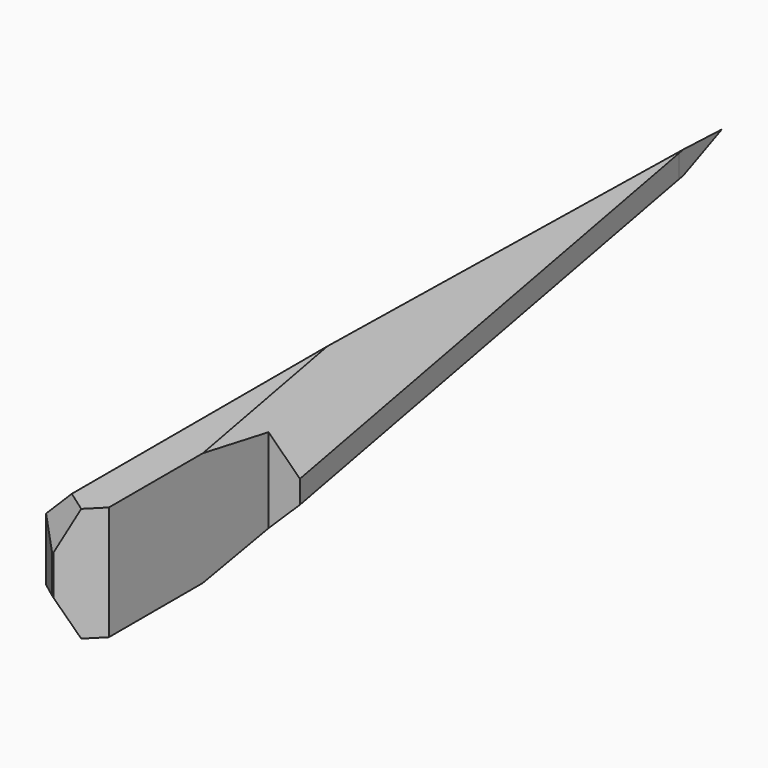
from build123d import *

# Parameters (mm, degrees)
F1_DEPTH     = 25.4
F2_SIZE      = 12.69999
F3_T1_DEPTH  = 188.8441409877
F4_DEPTH     = 20.574
F5_T1_DEPTH  = 49.2316398108
F5_T3_DEPTH  = 43.3636113916
F5_T5_DEPTH  = 43.3636113916
F5_T7_DEPTH  = 60.6732038629
F5_T12_DEPTH = 43.5108377847
F5_T17_DEPTH = 43.5108377847
F5_T22_DEPTH = 43.5108377847
F5_T27_DEPTH = 43.5108377847


# Not quite as in the source:
# - a fillet or chamfer that OpenCascade refuses, or shapes differently, is made with other operations: its cross-section is extruded or revolved along the edge and cut away or added
# - a fillet or chamfer is up to 0.001 mm smaller than in the source, because OpenCascade refuses the exact size


with BuildPart() as f1:
    # F0 (on Top) → F1 (new body)
    with BuildSketch(Plane.XY):
        Polygon((-6.9792079739, 0), (0, 0), (6.9792079739, 0), (13.9584159479, 0), (0, 76.0870501399), (-11.1239045018, 136.72323427), (-13.9584159479, 152.1741002798), (-13.9584159479, 76.0870501399), (-13.9584159479, 0), align=None)
        Polygon((6.9792079739, 0), (0, 0), (-6.9792079739, 0), (-6.9792079739, -30.6587181985), (-4.935038276, -30.6587181985), (6.9792079739, -30.6587181985), align=None)
    extrude(amount=F1_DEPTH)

    # F2 (size 12.7 in the source; OpenCascade refuses exactly that, so slightly less here)
    f2_edges = [f1.edges().sort_by_distance(p)[0] for p in [
        (-13.958416, 76.08705, 25.4),
        (-13.958416, 76.08705, 0),
    ]]
    chamfer(f2_edges, length=F2_SIZE)

    # F3: chamfer of 10.16 on 2 edges, made by hand

    # F3_s2 → F3_t1 (cut)
    with BuildSketch(Plane(origin=(5.1691181491, -28.1767611209, 0), x_dir=(0, 0, 1), z_dir=(-0.1804419719, 0.9835856316, 0))):
        Polygon((15.24, 13.7292973667), (25.4, 3.5692973667), (25.4, 13.7292973667), align=None)
        Polygon((10.16, 13.7292973667), (0, 3.5692973667), (0, 13.7292973667), align=None)
    extrude(amount=F3_T1_DEPTH, mode=Mode.SUBTRACT)

    # F4 (add): a face of the model
    f4_faces = [f1.faces().sort_by_distance(p)[0] for p in [
        (0.5158291465, -30.6587181985, 12.7),
    ]]
    extrude(f4_faces, amount=F4_DEPTH)

    # F5: chamfer of 6.858 on 6 edges, made by hand

    # F5_s2 → F5_t1 (cut)
    with BuildSketch(Plane.XY.offset(-11.9158199054)):
        Polygon((-0.1212079739, -51.2327181985), (-6.9792079739, -44.3747181985), (-6.9792079739, -51.2327181985), align=None)
    extrude(amount=F5_T1_DEPTH, mode=Mode.SUBTRACT)

    # F5_s4 → F5_t3 (cut)
    with BuildSketch(Plane(origin=(-18.8209558228, 0, 18.8209558228), x_dir=(0, 1, 0), z_dir=(0.7071067812, 0, -0.7071067812))):
        Polygon((-51.2327181985, 5.9681584787), (-44.3747181985, -0.8898415213), (-51.2327181985, -0.8898415213), align=None)
    extrude(amount=F5_T3_DEPTH, mode=Mode.SUBTRACT)

    # F5_s6 → F5_t5 (cut)
    with BuildSketch(Plane(origin=(-6.1209558228, 0, -6.1209558228), x_dir=(0, 1, 0), z_dir=(0.7071067812, 0, 0.7071067812))):
        Polygon((-51.2327181985, 11.9923537635), (-44.3747181985, 18.8503537635), (-51.2327181985, 18.8503537635), align=None)
    extrude(amount=F5_T5_DEPTH, mode=Mode.SUBTRACT)

    # F5_s8 → F5_t7 (cut)
    with BuildSketch(Plane.XY.offset(-17.6366019315)):
        Polygon((0.1212079739, -51.2327181985), (6.9792079739, -44.3747181985), (6.9792079739, -51.2327181985), align=None)
    extrude(amount=F5_T7_DEPTH, mode=Mode.SUBTRACT)


with BuildPart() as f5_tool10:
    # F5_s11 → F5_t12 (new body)
    with BuildSketch(Plane.YZ.offset(-18.8950278793)):
        Polygon((-51.2327181985, 6.858), (-44.3747181985, 0), (-51.2327181985, 0), align=None)
    extrude(amount=F5_T12_DEPTH)

    split(bisect_by=Plane(origin=(-16.0034385627, -22.6322798599, -16.0034385627), x_dir=(0.8164965809, -0.5773502692, 0), z_dir=(-0.5, -0.7071067812, -0.5)), keep=Keep.TOP)


with BuildPart() as f1_1:
    add(f1.part)

    # F5_t9: cut F5_tool10
    add(f5_tool10.part, mode=Mode.SUBTRACT)


with BuildPart() as f5_tool15:
    # F5_s16 → F5_t17 (new body)
    with BuildSketch(Plane.YZ.offset(-18.8950278793)):
        Polygon((-51.2327181985, 6.858), (-44.3747181985, 0), (-51.2327181985, 0), align=None)
    extrude(amount=F5_T17_DEPTH)

    split(bisect_by=Plane(origin=(25.6769630862, -25.6769630862, 0), x_dir=(0, 0, 1), z_dir=(0.7071067812, -0.7071067812, 0)), keep=Keep.TOP)


with BuildPart() as f1_2:
    add(f1_1.part)

    # F5_t14: cut F5_tool15
    add(f5_tool15.part, mode=Mode.SUBTRACT)


with BuildPart() as f5_tool20:
    # F5_s21 → F5_t22 (new body)
    with BuildSketch(Plane.YZ.offset(-18.8950278793)):
        Polygon((-44.3747181985, 25.4), (-51.2327181985, 18.542), (-51.2327181985, 25.4), align=None)
    extrude(amount=F5_T22_DEPTH)

    split(bisect_by=Plane(origin=(-22.3534385627, -31.612535981, 22.3534385627), x_dir=(0.8164965809, -0.5773502692, 0), z_dir=(-0.5, -0.7071067812, 0.5)), keep=Keep.TOP)


with BuildPart() as f1_3:
    add(f1_2.part)

    # F5_t19: cut F5_tool20
    add(f5_tool20.part, mode=Mode.SUBTRACT)


with BuildPart() as f5_tool25:
    # F5_s26 → F5_t27 (new body)
    with BuildSketch(Plane.YZ.offset(-18.8950278793)):
        Polygon((-44.3747181985, 25.4), (-51.2327181985, 18.542), (-51.2327181985, 25.4), align=None)
    extrude(amount=F5_T27_DEPTH)

    split(bisect_by=Plane(origin=(25.6769630862, -25.6769630862, 0), x_dir=(0, 0, 1), z_dir=(0.7071067812, -0.7071067812, 0)), keep=Keep.TOP)


with BuildPart() as f1_4:
    add(f1_3.part)

    # F5_t24: cut F5_tool25
    add(f5_tool25.part, mode=Mode.SUBTRACT)


solid = f1_4.part
